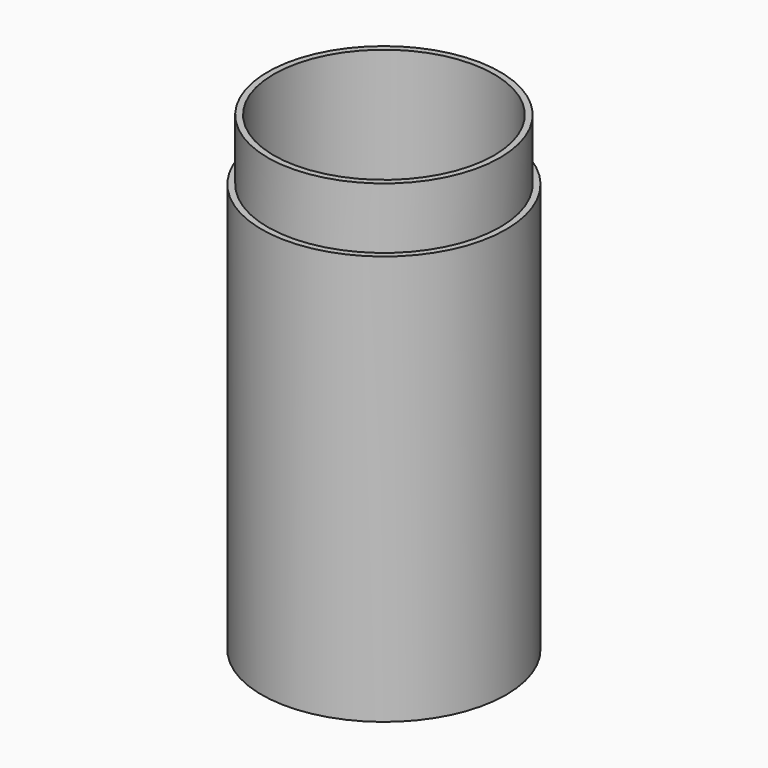
from build123d import *

# Parameters (mm, degrees)
F0_R     = 20
F1_DEPTH = 2
F2_R     = 20
F2_R_2   = 18
F3_DEPTH = 75
F4_R     = 20
F4_R_2   = 19
F5_DEPTH = 10


with BuildPart() as f1:
    # F0 (on Top) → F1 (new body)
    with BuildSketch(Plane.XY):
        Circle(F0_R)
    extrude(amount=F1_DEPTH)

    # F2 (on face) → F3 (join)
    with BuildSketch(Plane.XY.offset(2)):
        Circle(F2_R)
        Circle(F2_R_2, mode=Mode.SUBTRACT)
    extrude(amount=F3_DEPTH)

    # F4 (on face) → F5 (cut)
    with BuildSketch(Plane.XY.offset(77)):
        Circle(F4_R)
        Circle(F4_R_2, mode=Mode.SUBTRACT)
    extrude(amount=-F5_DEPTH, mode=Mode.SUBTRACT)


solid = f1.part
